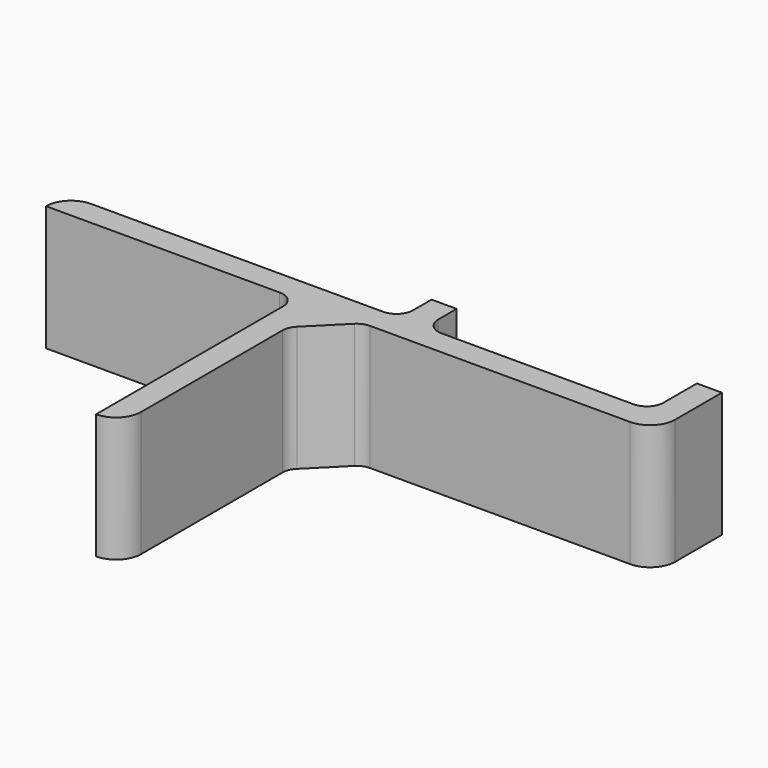
from build123d import *

# Parameters (mm, degrees)
F0_W     = 30
F0_H     = 3
F0_W_2   = 3
F0_H_2   = 4.7552157193
F0_H_3   = 7
F1_DEPTH = 15
F2_R     = 2
F3_SIZE  = 5
F4_R     = 2
F5_R     = 3
F6_R     = 2.99999
F7_R     = 2.99999
F8_R     = 2
F9_R     = 2


# Not quite as in the source:
# - a fillet or chamfer is up to 0.001 mm smaller than in the source, because OpenCascade refuses the exact size


with BuildPart() as f1:
    # F0 (on Top) → F1 (new body)
    with BuildSketch(Plane.XY):
        with Locations((-15, -1.5)):
            Rectangle(F0_W, F0_H)
        Polygon((3, 0), (0, 0), (0, -3), (0, -33), (3, -33), (3, -3), align=None)
        Polygon((10, 0), (3, 0), (3, -3), (43, -3), (43, 0), (40, 0), (13, 0), align=None)
        with Locations((11.5, 2.3776078597)):
            Rectangle(F0_W_2, F0_H_2)
        with Locations((41.5, 3.5)):
            Rectangle(F0_W_2, F0_H_3)
    extrude(amount=F1_DEPTH)

    # F2
    f2_edges = [f1.edges().sort_by_distance(p)[0] for p in [
        (0, -3, 7.5),
    ]]
    fillet(f2_edges, radius=F2_R)

    # F3
    f3_edges = [f1.edges().sort_by_distance(p)[0] for p in [
        (3, -3, 7.5),
    ]]
    chamfer(f3_edges, length=F3_SIZE)

    # F4
    f4_edges = [f1.edges().sort_by_distance(p)[0] for p in [
        (13, 0, 7.5),
        (40, 0, 7.5),
        (10, 0, 7.5),
    ]]
    fillet(f4_edges, radius=F4_R)

    # F5
    f5_edges = [f1.edges().sort_by_distance(p)[0] for p in [
        (43, -3, 7.5),
    ]]
    fillet(f5_edges, radius=F5_R)

    # F6 (radius 3 in the source; OpenCascade refuses exactly that, so slightly less here)
    f6_edges = [f1.edges().sort_by_distance(p)[0] for p in [
        (-30, 0, 7.5),
    ]]
    fillet(f6_edges, radius=F6_R)

    # F7 (radius 3 in the source; OpenCascade refuses exactly that, so slightly less here)
    f7_edges = [f1.edges().sort_by_distance(p)[0] for p in [
        (3, -33, 7.5),
    ]]
    fillet(f7_edges, radius=F7_R)

    # F8
    f8_edges = [f1.edges().sort_by_distance(p)[0] for p in [
        (8, -3, 7.5),
    ]]
    fillet(f8_edges, radius=F8_R)

    # F9
    f9_edges = [f1.edges().sort_by_distance(p)[0] for p in [
        (3, -8, 7.5),
    ]]
    fillet(f9_edges, radius=F9_R)


solid = f1.part
